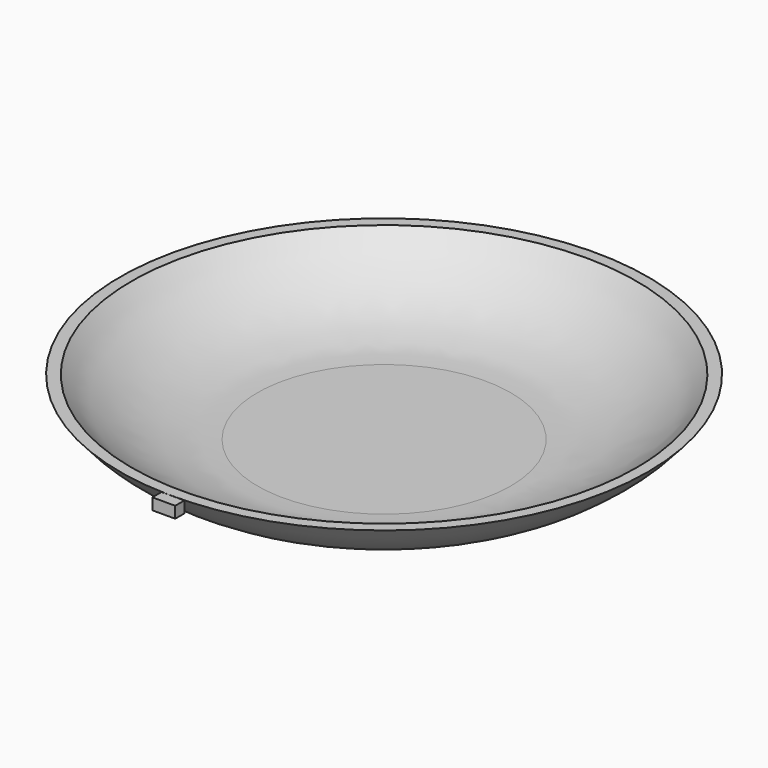
from build123d import *

# Parameters (mm, degrees)
F0_R     = 76.2
F1_DEPTH = 19.05
F3_T     = -2.54
F5_DEPTH = 3.302


# Not quite as in the source:
# - a fillet or chamfer that OpenCascade refuses, or shapes differently, is made with other operations: its cross-section is extruded or revolved along the edge and cut away or added
# - a feature names something its author has since deleted; it is built from what else it names


with BuildPart() as f1:
    # F0 (on Top) → F1 (new body)
    with BuildSketch(Plane.XY):
        Circle(F0_R)
    extrude(amount=F1_DEPTH)

    # F2: fillet of radius 50.8 on 1 edges, made by hand

    # F2_s1 → F2_t2 (revolve, cut)
    with BuildSketch(Plane.XZ):
        with BuildLine():
            ThreePointArc((76.2, 19.05), (58.5413079663, 5.0094988016), (36.5442627102, 0))
            Line((36.5442627102, 0), (76.2, 0))
            Line((76.2, 0), (76.2, 19.05))
        make_face()
    revolve(axis=Axis((0, 0, 0), (0, 0, 1)), mode=Mode.SUBTRACT)

    # F3
    f3_openings = [f1.faces().sort_by_distance(p)[0] for p in [
        (0, 0, 19.05),
    ]]
    offset(amount=F3_T, openings=f3_openings)


with BuildPart() as f5:
    # F4 (on face) → F5 (new body)
    with BuildSketch(Plane.XY.offset(19.05)):
        Polygon((3.302, -76.2), (0, -76.2), (-3.302, -76.2), (-3.302, -79.502), (3.302, -79.502), align=None)
    extrude(amount=-F5_DEPTH)


solid = Compound([f1.part, f5.part])
